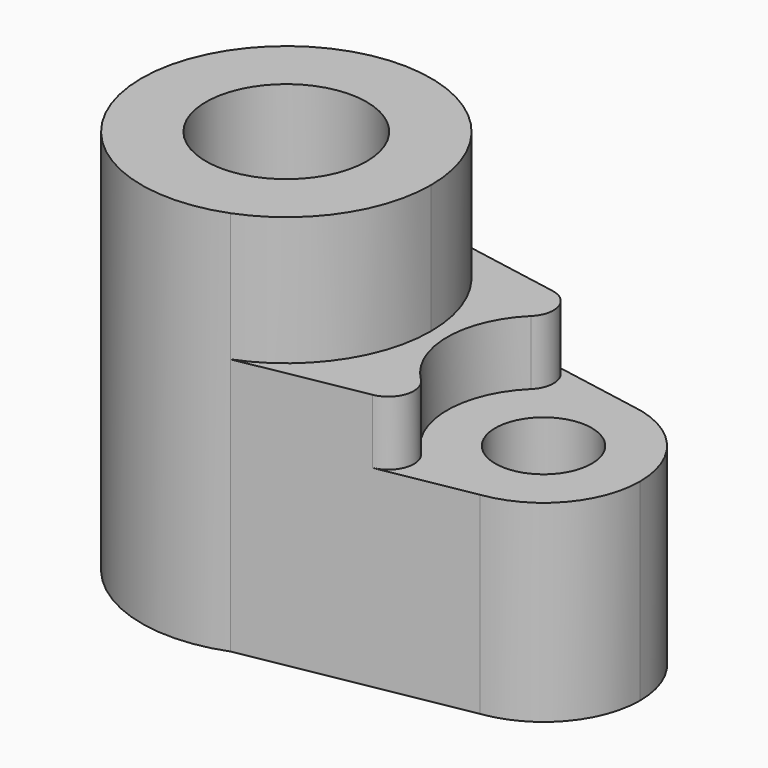
from build123d import *
from build123d import SkipClean  # not in build123d's __all__

# Parameters (mm, degrees)
F0_R     = 15.875
F0_R_2   = 9.525
F1_DEPTH = 76.2
F2_DEPTH = 38.1
F3_DEPTH = 25.4
F4_R     = 5.08


with BuildPart() as f1:
    # F0 (on Top) → F1 (new body)
    with BuildSketch(Plane.XY):
        with BuildLine():
            ThreePointArc((10.3219202517, 26.6456110329), (23.5741330296, 16.1490209271), (28.575, 0))
            ThreePointArc((28.575, 0), (23.5741330296, -16.1490209271), (10.3219202517, -26.6456110329))
            Line((10.3219202517, -26.6456110329), (53.34, -18.8799073091))
            ThreePointArc((53.34, -18.8799073091), (31.75, 0), (53.34, 18.8799073091))
            Line((53.34, 18.8799073091), (10.3219202517, 26.6456110329))
        make_face()
        with BuildLine():
            ThreePointArc((10.3219202517, -26.6456110329), (23.5741330296, -16.1490209271), (28.575, 0))
            ThreePointArc((28.575, 0), (23.5741330296, 16.1490209271), (10.3219202517, 26.6456110329))
            ThreePointArc((10.3219202517, 26.6456110329), (-28.575, 0), (10.3219202517, -26.6456110329))
        make_face()
        Circle(F0_R, mode=Mode.SUBTRACT)
        with BuildLine():
            ThreePointArc((69.85, 0), (65.1403190341, 12.5402452129), (53.34, 18.8799073091))
            ThreePointArc((53.34, 18.8799073091), (31.75, 0), (53.34, -18.8799073091))
            ThreePointArc((53.34, -18.8799073091), (65.1403190341, -12.5402452129), (69.85, 0))
        make_face()
        with Locations((50.8, 0)):
            Circle(F0_R_2, mode=Mode.SUBTRACT)
    extrude(amount=-F1_DEPTH)

    # F0 (on Top) → F2 (cut)
    with BuildSketch(Plane.XY):
        with BuildLine():
            ThreePointArc((69.85, 0), (65.1403190341, 12.5402452129), (53.34, 18.8799073091))
            ThreePointArc((53.34, 18.8799073091), (31.75, 0), (53.34, -18.8799073091))
            ThreePointArc((53.34, -18.8799073091), (65.1403190341, -12.5402452129), (69.85, 0))
        make_face()
        with Locations((50.8, 0)):
            Circle(F0_R_2, mode=Mode.SUBTRACT)
    extrude(amount=-F2_DEPTH, mode=Mode.SUBTRACT)

    # F0 (on Top) → F3 (cut)
    with BuildSketch(Plane.XY):
        with BuildLine():
            ThreePointArc((10.3219202517, 26.6456110329), (23.5741330296, 16.1490209271), (28.575, 0))
            ThreePointArc((28.575, 0), (23.5741330296, -16.1490209271), (10.3219202517, -26.6456110329))
            Line((10.3219202517, -26.6456110329), (53.34, -18.8799073091))
            ThreePointArc((53.34, -18.8799073091), (31.75, 0), (53.34, 18.8799073091))
            Line((53.34, 18.8799073091), (10.3219202517, 26.6456110329))
        make_face()
    with SkipClean():  # cleaning this boolean's faces spoils the solid; the shape is the same uncleaned
        extrude(amount=-F3_DEPTH, mode=Mode.SUBTRACT)

    # F4
    f4_edges = [f1.edges().sort_by_distance(p)[0] for p in [
        (53.34, -18.879907, -31.75),
        (53.34, -18.879907, -57.15),
        (53.34, 18.879907, -31.75),
        (53.34, 18.879907, -57.15),
    ]]
    fillet(f4_edges, radius=F4_R)


solid = f1.part
